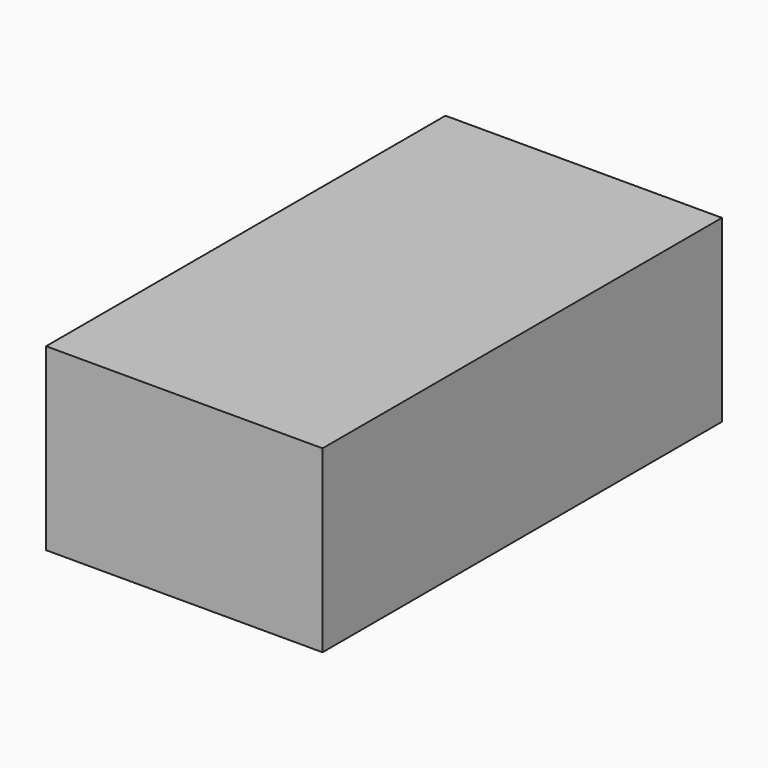
from build123d import *

# Parameters (mm, degrees)
F2_W     = 39.1040146351
F2_H     = 70.6124361604
F3_DEPTH = 25.4


# Not quite as in the source:
# - the program builds the solid bodies; features that only make, move or delete a surface that nothing else refers to are left out


with BuildPart() as f3:
    # F2 (on Top) → F3 (new body)
    with BuildSketch(Plane.XY):
        with Locations((113.580390811, 8.9965434745)):
            Rectangle(F2_W, F2_H)
    extrude(amount=F3_DEPTH)


solid = f3.part
